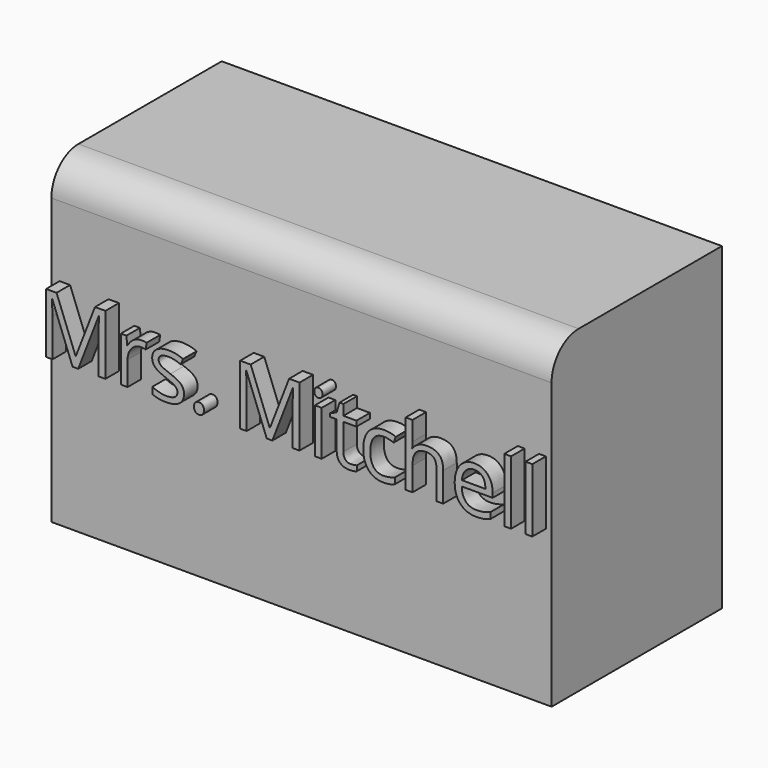
from build123d import *

# Parameters (mm, degrees)
F0_W         = 75.1867033541
F0_H         = 47.9492582381
F1_DEPTH     = 32.004
F2_T         = -2.54
F3_R         = 5.08
F4_TEXT_SIZE = 12.6099265698
F5_DEPTH     = 34.544


# Not quite as in the source:
# - Text() gives the source's letters only with a copy of the font that has no kerning and outlines rounded to 1/6400 em; it was checked with that copy


with BuildPart() as f1:
    # F0 (on Front) → F1 (new body)
    with BuildSketch(Plane.XZ):
        with Locations((-2.127924934, 23.974629119)):
            Rectangle(F0_W, F0_H)
    extrude(amount=F1_DEPTH)

    # F2
    f2_openings = [f1.faces().sort_by_distance(p)[0] for p in [
        (-2.127925, -16.002, 0),
    ]]
    offset(amount=F2_T, openings=f2_openings)

    # F3
    f3_edges = [f1.edges().sort_by_distance(p)[0] for p in [
        (-2.127925, -32.004, 47.949258),
    ]]
    fillet(f3_edges, radius=F3_R)

    # F4 (on Front) → F5 (join)
    with BuildSketch(Plane.XZ):
        with Locations((-39.7212784737, 23.2653208077)):
            Text('Mrs. Mitchell', F4_TEXT_SIZE, font='Open Sans', text_align=(TextAlign.LEFT, TextAlign.BOTTOM))
    extrude(amount=F5_DEPTH)


solid = f1.part
